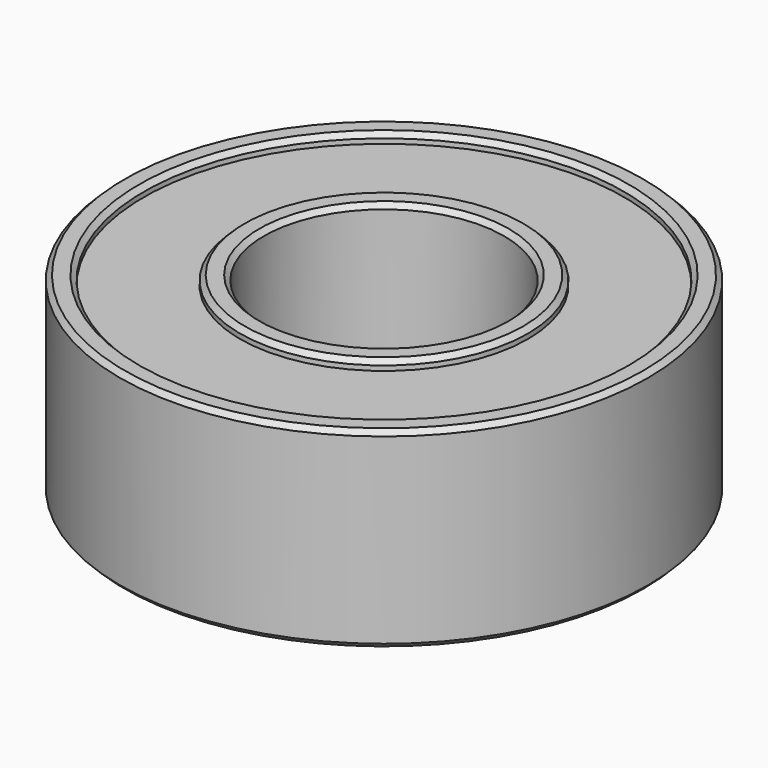
from build123d import *

# Parameters (mm, degrees)
F0_R     = 3
F0_R_2   = 2.5
F1_DEPTH = 4
F0_R_3   = 5.5
F0_R_4   = 5
F2_START = 0.2
F2_DEPTH = 3.6
F3_SIZE  = 0.1


with BuildPart() as f1:
    # F0 (on Top) → F1 (new body)
    with BuildSketch(Plane.XY):
        Circle(F0_R)
        Circle(F0_R_2, mode=Mode.SUBTRACT)
    extrude(amount=F1_DEPTH)



with BuildPart() as f1b:
    # F0 (on Top) → F1, piece 2 (new body)
    with BuildSketch(Plane.XY):
        Circle(F0_R_3)
        Circle(F0_R_4, mode=Mode.SUBTRACT)
    extrude(amount=F1_DEPTH)


with BuildPart() as f1_1:
    add(f1.part)

    add(f1b.part)  # F2 merges F1b
    # F0 (on Top) → F2 (join)
    with BuildSketch(Plane.XY.offset(F2_START)):
        Circle(F0_R_4)
        Circle(F0_R, mode=Mode.SUBTRACT)
    extrude(amount=F2_DEPTH)

    # F3
    f3_edges = [f1_1.edges().sort_by_distance(p)[0] for p in [
        (-3, 0, 0),
        (-2.5, 0, 0),
        (-5.5, 0, 4),
        (-5, 0, 4),
        (-3, 0, 4),
        (-2.5, 0, 4),
        (-5.5, 0, 0),
        (-5, 0, 0),
    ]]
    chamfer(f3_edges, length=F3_SIZE)


solid = f1_1.part
